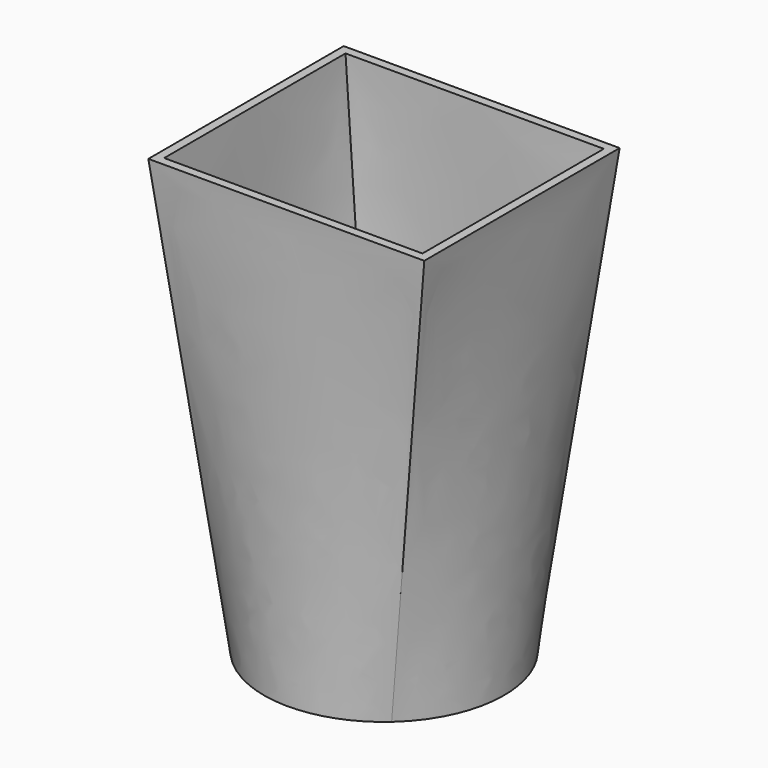
from build123d import *

# Parameters (mm, degrees)
F2_W = 80.009996891
F2_H = 70.8002150059
F4_T = 2.54


# Not quite as in the source:
# - the arcs of a loft's sections are written as splines that run evenly, so that the points pair up as in the source's solid
# - a shell that OpenCascade refuses in one call is made with other operations: the cavity is built on its own and cut out


with BuildPart() as f3:
    # F2 (on offset) → F3 section 0
    with BuildSketch(Plane.XY.offset(127)):
        Rectangle(F2_W, F2_H)
    # F0 (on Top) → F3 section 1
    with BuildSketch(Plane.XY):
        with BuildLine():
            add(Edge.make_bspline(
                [(26.065590987, 23.0652358186), (24.5559748328, 24.7712247593), (22.8783749167, 26.3284909791), (19.2515124469, 29.085885659), (17.3023395745, 30.2859459372), (13.2072252341, 32.2827922844), (11.0613850258, 33.0795289775), (6.6553917622, 34.2390893068), (4.3953476538, 34.6018842705), (-0.1522046827, 34.8795973285), (-2.4396004636, 34.7945085558), (-6.953951987, 34.1797019856), (-9.1807961033, 33.6499993904), (-13.4884628163, 32.1662998637), (-15.5691788974, 31.2123396195), (-19.5046195839, 28.916764877), (-21.3592468778, 27.5752071412), (-23.0652358186, 26.065590987)],
                knots=[0, 0, 0, 0, 0.125, 0.125, 0.25, 0.25, 0.375, 0.375, 0.5, 0.5, 0.625, 0.625, 0.75, 0.75, 0.875, 0.875, 1, 1, 1, 1], degree=3))
            add(Edge.make_bspline(
                [(-23.0652358186, 26.065590987), (-24.7712247593, 24.5559748328), (-26.3284909791, 22.8783749167), (-29.085885659, 19.2515124469), (-30.2859459372, 17.3023395745), (-32.2827922844, 13.2072252341), (-33.0795289775, 11.0613850258), (-34.2390893068, 6.6553917622), (-34.6018842705, 4.3953476538), (-34.8795973285, -0.1522046827), (-34.7945085558, -2.4396004636), (-34.1797019856, -6.953951987), (-33.6499993904, -9.1807961033), (-32.1662998637, -13.4884628163), (-31.2123396195, -15.5691788974), (-28.916764877, -19.5046195839), (-27.5752071412, -21.3592468778), (-26.065590987, -23.0652358186)],
                knots=[0, 0, 0, 0, 0.125, 0.125, 0.25, 0.25, 0.375, 0.375, 0.5, 0.5, 0.625, 0.625, 0.75, 0.75, 0.875, 0.875, 1, 1, 1, 1], degree=3))
            add(Edge.make_bspline(
                [(-26.065590987, -23.0652358186), (-24.5559748328, -24.7712247593), (-22.8783749167, -26.3284909791), (-19.2515124469, -29.085885659), (-17.3023395745, -30.2859459372), (-13.2072252341, -32.2827922844), (-11.0613850258, -33.0795289775), (-6.6553917622, -34.2390893068), (-4.3953476538, -34.6018842705), (0.1522046827, -34.8795973285), (2.4396004636, -34.7945085558), (6.953951987, -34.1797019856), (9.1807961033, -33.6499993904), (13.4884628163, -32.1662998637), (15.5691788974, -31.2123396195), (19.5046195839, -28.916764877), (21.3592468778, -27.5752071412), (23.0652358186, -26.065590987)],
                knots=[0, 0, 0, 0, 0.125, 0.125, 0.25, 0.25, 0.375, 0.375, 0.5, 0.5, 0.625, 0.625, 0.75, 0.75, 0.875, 0.875, 1, 1, 1, 1], degree=3))
            add(Edge.make_bspline(
                [(23.0652358186, -26.065590987), (24.7712247593, -24.5559748328), (26.3284909791, -22.8783749167), (29.085885659, -19.2515124469), (30.2859459372, -17.3023395745), (32.2827922844, -13.2072252341), (33.0795289775, -11.0613850258), (34.2390893068, -6.6553917622), (34.6018842705, -4.3953476538), (34.8795973285, 0.1522046827), (34.7945085558, 2.4396004636), (34.1797019856, 6.953951987), (33.6499993904, 9.1807961033), (32.1662998637, 13.4884628163), (31.2123396195, 15.5691788974), (28.916764877, 19.5046195839), (27.5752071412, 21.3592468778), (26.065590987, 23.0652358186)],
                knots=[0, 0, 0, 0, 0.125, 0.125, 0.25, 0.25, 0.375, 0.375, 0.5, 0.5, 0.625, 0.625, 0.75, 0.75, 0.875, 0.875, 1, 1, 1, 1], degree=3))
        make_face()
    loft(ruled=True)

    # F4: shell of thickness 2.54, made by hand


with BuildPart() as f4_core1:
    # F4_t2: copy of F3
    add(f3.part)

    # the walls: a layer under each face that stays
    f4_faces = [f4_core1.faces().sort_by_distance(p)[0] for p in [
        (37.3728696225, -1.0607857428, 63.5),
        (1.0607857428, 35.0704241512, 63.5),
        (-37.3728696225, 1.0607857428, 63.5),
        (-1.0607857428, -35.0704241512, 63.5),
        (0, 0, 0),
    ]]
    thicken(f4_faces, amount=-F4_T, mode=Mode.SUBTRACT)


with BuildPart() as f3_1:
    add(f3.part)

    # what is left inside the walls is the cavity
    f4_cavity = [f4_core1.part.solids().sort_by_distance(p)[0] for p in [
        (-0.656082, -32.618968, 85.395704),
    ]]
    add(f4_cavity, mode=Mode.SUBTRACT)


solid = f3_1.part
